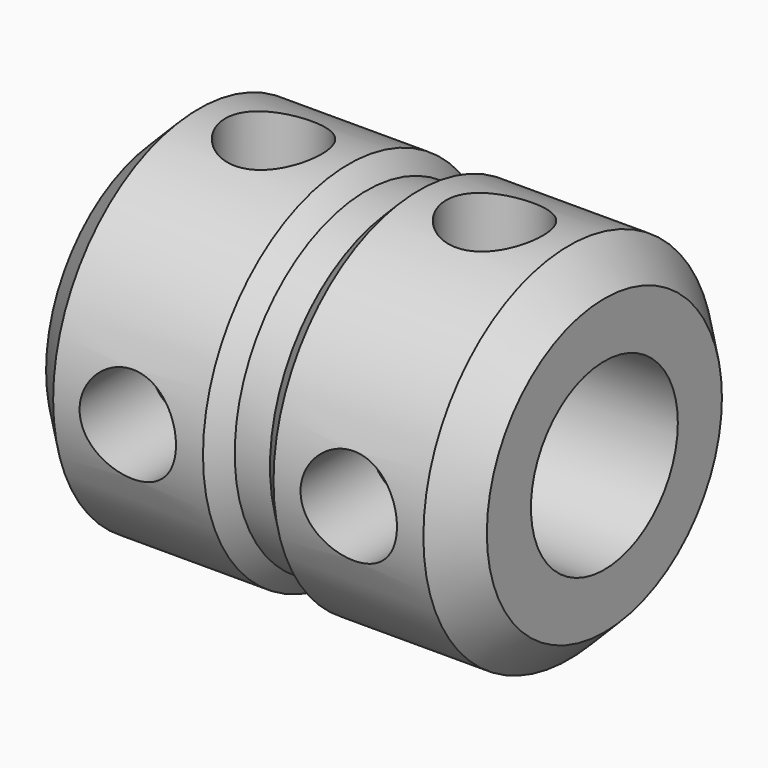
from build123d import *

# Parameters (mm, degrees)
F0_R          = 7.112
F1_DEPTH      = 0.762
F1_DEPTH_BACK = 0.762
F2_R          = 7.874
F2_R_2        = 7.112
F3_DEPTH      = 8.763
F4_R          = 7.874
F4_R_2        = 7.112
F5_DEPTH      = 8.763
F9_R          = 3.96875
F10_DEPTH     = 25.4
F8_R          = 2.0828
F11_DEPTH     = 7.62
F14_R         = 2.0828
F15_DEPTH     = 7.874
F16_SIZE      = 1.524
F17_SIZE      = 0.76199


# Not quite as in the source:
# - a fillet or chamfer is up to 0.001 mm smaller than in the source, because OpenCascade refuses the exact size
# - a pattern or mirror of a feature is missing from the dataset's text; its kind, count and spacing are read off the source's solid


with BuildPart() as f1:
    # F0 (on Right) → F1 (new body, two sides)
    with BuildSketch(Plane.YZ) as f1_sk:
        Circle(F0_R)
    extrude(amount=F1_DEPTH)
    extrude(f1_sk.sketch, amount=-F1_DEPTH_BACK)

    # F2 (on face) → F3 (join)
    with BuildSketch(Plane.YZ.offset(0.762)):
        Circle(F2_R)
        Circle(F2_R_2, mode=Mode.SUBTRACT)
        Circle(F2_R_2)
    f3 = extrude(amount=F3_DEPTH)

    # F3_copies: F3 across plane
    add(f3.mirror(Plane(origin=(0, 0, 0), x_dir=(0, 0, -1), z_dir=(-1, 0, 0))))

    # F4 (on face) → F5 (join)
    with BuildSketch(Plane(origin=(-0.762, 0, 0), x_dir=(0, -1, 0), z_dir=(-1, 0, 0))):
        Circle(F4_R)
        Circle(F4_R_2, mode=Mode.SUBTRACT)
    extrude(amount=F5_DEPTH)

    # F9 (on face) → F10 (cut)
    with BuildSketch(Plane.YZ.offset(9.525)):
        Circle(F9_R)
    extrude(amount=-F10_DEPTH, mode=Mode.SUBTRACT)

    # F8 (on plane+point) → F11 (cut)
    with BuildSketch(Plane.XY.offset(7.874)):
        with Locations((4.7752, 0)):
            Circle(F8_R)
        with Locations((-4.7752, 0)):
            Circle(F8_R)
    extrude(amount=-F11_DEPTH, mode=Mode.SUBTRACT)

    # F14 (on plane+point) → F15 (cut)
    with BuildSketch(Plane.XZ.offset(7.874)):
        with Locations((4.7752, 0)):
            Circle(F14_R)
        with Locations((-4.7752, 0)):
            Circle(F14_R)
    extrude(amount=-F15_DEPTH, mode=Mode.SUBTRACT)

    # F16
    f16_edges = [f1.edges().sort_by_distance(p)[0] for p in [
        (9.525, -7.874, 0),
        (-9.525, -7.874, 0),
    ]]
    chamfer(f16_edges, length=F16_SIZE)

    # F17 (size 0.762 in the source; OpenCascade refuses exactly that, so slightly less here)
    f17_edges = [f1.edges().sort_by_distance(p)[0] for p in [
        (0.762, -7.874, 0),
        (-0.762, -7.874, 0),
    ]]
    chamfer(f17_edges, length=F17_SIZE)


solid = f1.part
